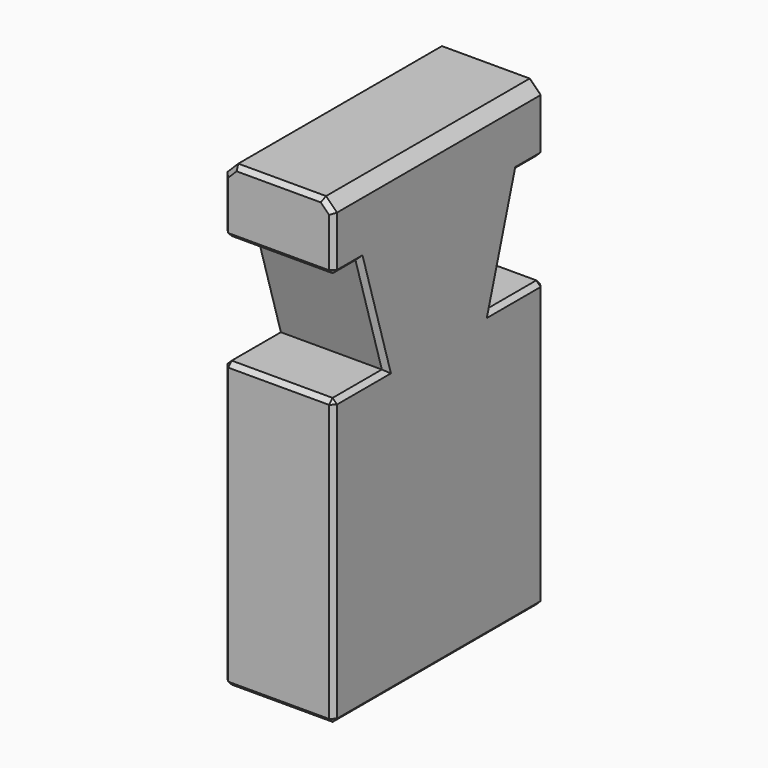
from build123d import *

# Parameters (mm, degrees)
F0_W          = 304.8
F0_H          = 533.4
F1_DEPTH      = 63.5
F1_DEPTH_BACK = 63.5
F3_DEPTH      = 127
F4_SIZE       = 12.7
F5_SIZE       = 5.08


# Not quite as in the source:
# - a feature names something its author has since deleted; it is built from what else it names


with BuildPart() as f1:
    # F0 (on Right) → F1 (new body, two sides)
    with BuildSketch(Plane.YZ) as f1_sk:
        Rectangle(F0_W, F0_H)
    extrude(amount=F1_DEPTH)
    extrude(f1_sk.sketch, amount=-F1_DEPTH_BACK)

    # F2 (on face) → F3 (cut, through all)
    with BuildSketch(Plane.YZ.offset(63.5)):
        Polygon((-114.3, 190.5), (-152.4, 190.5), (-152.4, 63.5), (-76.2, 63.5), align=None)
        Polygon((152.4, 190.5), (114.3, 190.5), (76.2, 63.5), (152.4, 63.5), align=None)
    extrude(amount=-F3_DEPTH, mode=Mode.SUBTRACT)

    # F4
    f4_edges = [f1.edges().sort_by_distance(p)[0] for p in [
        (63.5, 0, 266.7),
        (-63.5, 0, 266.7),
    ]]
    chamfer(f4_edges, length=F4_SIZE)

    # F5
    f5_edges = [f1.edges().sort_by_distance(p)[0] for p in [
        (63.5, -114.3, 63.5),
        (63.5, -95.25, 127),
        (63.5, -133.35, 190.5),
        (63.5, -152.4, 222.25),
        (57.15, -152.4, 260.35),
        (0, -152.4, 266.7),
        (-63.5, -152.4, 222.25),
        (0, -152.4, 190.5),
        (0, -152.4, 63.5),
        (-63.5, -114.3, 63.5),
        (-63.5, -95.25, 127),
        (-63.5, -133.35, 190.5),
        (-57.15, -152.4, 260.35),
        (-63.5, -152.4, -101.6),
        (0, -152.4, -266.7),
        (63.5, -152.4, -101.6),
        (-63.5, 0, -266.7),
        (63.5, 0, -266.7),
        (0, 152.4, -266.7),
        (63.5, 152.4, -101.6),
        (63.5, 114.3, 63.5),
        (63.5, 95.25, 127),
        (63.5, 133.35, 190.5),
        (63.5, 152.4, 222.25),
        (57.15, 152.4, 260.35),
        (0, 152.4, 266.7),
        (-57.15, 152.4, 260.35),
        (-63.5, 152.4, 222.25),
        (-63.5, 133.35, 190.5),
        (-63.5, 95.25, 127),
        (0, 152.4, 190.5),
        (-63.5, 114.3, 63.5),
        (0, 152.4, 63.5),
        (-63.5, 152.4, -101.6),
    ]]
    chamfer(f5_edges, length=F5_SIZE)


solid = f1.part
